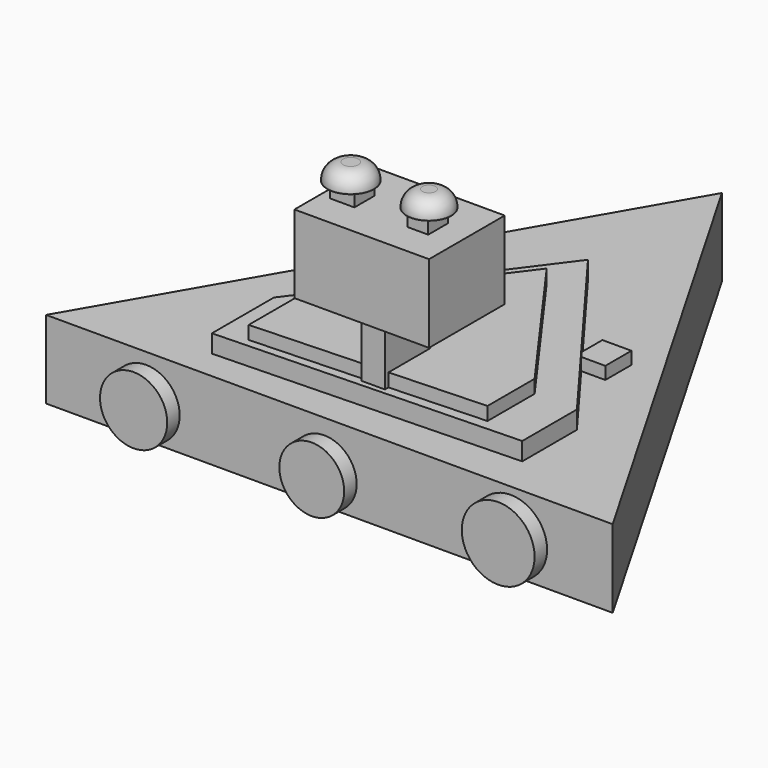
from build123d import *

# Parameters (mm, degrees)
F1_DEPTH  = 25.4
F2_W      = 7.7060335316
F2_H      = 18.2289350778
F3_DEPTH  = 25.4
F4_W      = 43.813964352
F4_H      = 30.7902917266
F5_DEPTH  = 25.4
F7_DEPTH  = 5.842
F9_DEPTH  = 4.318
F10_R     = 10.9377694976
F11_DEPTH = 5.08
F10_R_2   = 10.5571366777
F10_R_3   = 11.8519516329
F12_W     = 11.5590882488
F12_H     = 24.0346593782
F13_DEPTH = 3.048
F14_R     = 14.3871232907
F15_DEPTH = 4.318
F17_W     = 24.5277062058
F17_H     = 7.1590915322
F18_DEPTH = 1.778
F19_W     = 8.0961622298
F19_H     = 9.2830331996
F19_W_2   = 9.4388686121
F19_H_2   = 10.6246345676
F20_DEPTH = 4.064
F21_W     = 6.7095533013
F21_H     = 8.0418605357
F22_DEPTH = 4.826
F21_W_2   = 7.9630683176
F21_H_2   = 8.0924835056
F23_R     = 7.24746932
F24_DEPTH = 5.334
F23_R_2   = 7.57353882
F25_R     = 5.08
F26_R     = 5.08


# Not quite as in the source:
# - a fillet or chamfer that OpenCascade refuses, or shapes differently, is made with other operations: its cross-section is extruded or revolved along the edge and cut away or added


with BuildPart() as f1:
    # F0 (on Top) → F1 (new body)
    with BuildSketch(Plane.XY):
        Polygon((-92.2177294153, -53.241930902), (92.2177294153, -53.241930902), (0, 106.483861804), align=None)
    extrude(amount=F1_DEPTH)

    # F2 (on face) → F3 (join)
    with BuildSketch(Plane.XY.offset(25.4)):
        with Locations((3.8530167658, -31.1447037384)):
            Rectangle(F2_W, F2_H)
    extrude(amount=F3_DEPTH)

    # F4 (on face) → F5 (join)
    with BuildSketch(Plane.XY.offset(50.8)):
        with Locations((3.692750819, -29.2946621776)):
            Rectangle(F4_W, F4_H)
    extrude(amount=F5_DEPTH)

    # F6 (on face) → F7 (join)
    with BuildSketch(Plane.XY.offset(25.4)):
        Polygon((-45.9667816758, -43.5710027814), (52.6651255786, -40.6033433974), (52.6651255786, -18.3600392193), (3.388244193, 47.7468930185), (-45.9667816758, -18.3600392193), align=None)
    extrude(amount=F7_DEPTH)

    # F8 (on face) → F9 (join)
    with BuildSketch(Plane.XY.offset(31.242)):
        Polygon((-36.3797843456, -40.6033433974), (38.902554661, -37.5404730439), (38.902554661, -18.3600392193), (3.388244193, 30.9511683881), (-36.3797843456, -21.8821838498), align=None)
    extrude(amount=F9_DEPTH)

    # F14 (on face) → F15 (join)
    with BuildSketch(Plane(origin=(0, 0, 0), x_dir=(1, 0, 0), z_dir=(0, 0, -1))):
        with Locations((1.6217207303, -33.9718163013)):
            Circle(F14_R)
    extrude(amount=F15_DEPTH)

    # F16: fillet of radius 5.08 on 1 edges, made by hand

    # F16_s1 → F16_t2 (revolve, cut)
    with BuildSketch(Plane.XZ.offset(-33.9718163013)):
        with BuildLine():
            ThreePointArc((16.008844021, 0), (14.2980739798, -3.0901007256), (10.986319158, -4.318))
            Line((10.986319158, -4.318), (16.008844021, -4.318))
            Line((16.008844021, -4.318), (16.008844021, 0))
        make_face()
    revolve(axis=Axis((1.6217207303, 33.9718163013, -4.318), (0, 0, -1)), mode=Mode.SUBTRACT)

    # F19 (on face) → F20 (join)
    with BuildSketch(Plane.XY.offset(25.4)):
        with Locations((-38.2937844843, 17.7833898924)):
            Rectangle(F19_W, F19_H)
        with Locations((36.4500377327, 12.8823302221)):
            Rectangle(F19_W_2, F19_H_2)
    extrude(amount=F20_DEPTH)


with BuildPart() as f11:
    # F10 (on face) → F11 (new body)
    with BuildSketch(Plane.XZ.offset(53.241930902)):
        with Locations((-59.6596300602, 10.7411490753)):
            Circle(F10_R)
    extrude(amount=F11_DEPTH)


with BuildPart() as f11b:
    # F10 (on face) → F11, piece 2 (new body)
    with BuildSketch(Plane.XZ.offset(53.241930902)):
        with Locations((-1.674802741, 9.7942696884)):
            Circle(F10_R_2)
    extrude(amount=F11_DEPTH)


with BuildPart() as f11c:
    # F10 (on face) → F11, piece 3 (new body)
    with BuildSketch(Plane.XZ.offset(53.241930902)):
        with Locations((59.0170994401, 11.1700361595)):
            Circle(F10_R_3)
    extrude(amount=F11_DEPTH)


with BuildPart() as f13:
    # F12 (on face) → F13 (new body)
    with BuildSketch(Plane(origin=(0, 0, 0), x_dir=(1, 0, 0), z_dir=(0, 0, -1))):
        with Locations((-0.2612734679, 5.0718975253)):
            Rectangle(F12_W, F12_H)
    extrude(amount=F13_DEPTH)


with BuildPart() as f18:
    # F17 (on face) → F18 (new body)
    with BuildSketch(Plane(origin=(0, -13.8995163143, 0), x_dir=(-1, 0, 0), z_dir=(0, 1, 0))):
        with Locations((-1.7953896895, 65.8626444638)):
            Rectangle(F17_W, F17_H)
    extrude(amount=F18_DEPTH)


with BuildPart() as f22:
    # F21 (on face) → F22 (new body)
    with BuildSketch(Plane.XY.offset(76.2)):
        with Locations((13.6541202664, -30.2609531209)):
            Rectangle(F21_W, F21_H)
    extrude(amount=F22_DEPTH)


with BuildPart() as f22b:
    # F21 (on face) → F22, piece 2 (new body)
    with BuildSketch(Plane.XY.offset(76.2)):
        with Locations((-11.0076835845, -30.235641636)):
            Rectangle(F21_W_2, F21_H_2)
    extrude(amount=F22_DEPTH)


with BuildPart() as f24:
    # F23 (on face) → F24 (new body)
    with BuildSketch(Plane.XY.offset(81.026)):
        with Locations((13.6464145035, -29.7668650746)):
            Circle(F23_R)
    extrude(amount=F24_DEPTH)

    # F26
    f26_edges = [f24.edges().sort_by_distance(p)[0] for p in [
        (6.398945, -29.766865, 86.36),
    ]]
    fillet(f26_edges, radius=F26_R)


with BuildPart() as f24b:
    # F23 (on face) → F24, piece 2 (new body)
    with BuildSketch(Plane.XY.offset(81.026)):
        with Locations((-11.1858844757, -30.5551066995)):
            Circle(F23_R_2)
    extrude(amount=F24_DEPTH)

    # F25
    f25_edges = [f24b.edges().sort_by_distance(p)[0] for p in [
        (-18.759423, -30.555107, 86.36),
    ]]
    fillet(f25_edges, radius=F25_R)


solid = Compound([f1.part, f11.part, f11b.part, f11c.part, f13.part, f18.part, f22.part, f22b.part, f24.part, f24b.part])
